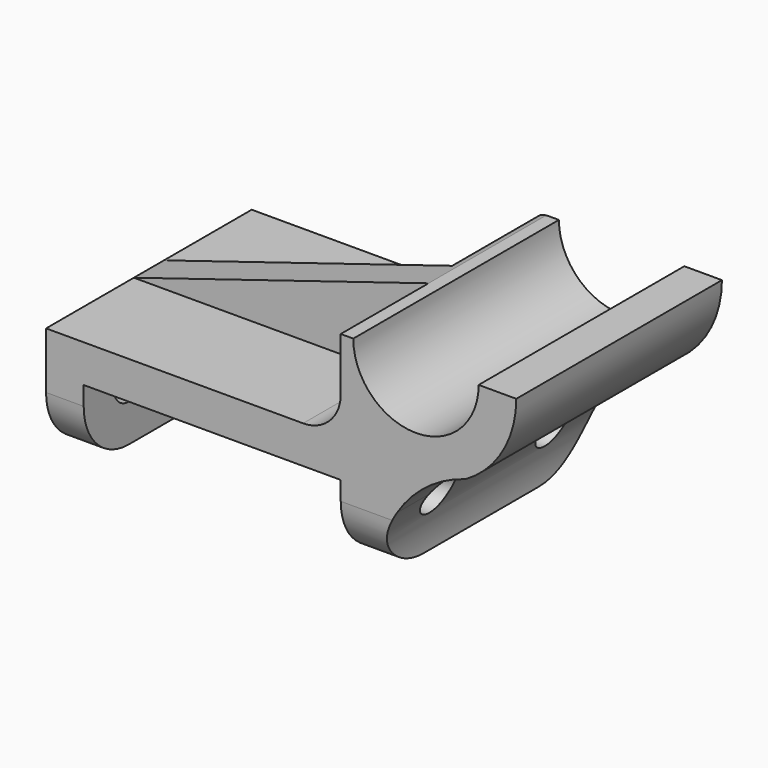
from build123d import *

# Parameters (mm, degrees)
F0_W      = 150
F0_H      = 65
F1_DEPTH  = 82
F10_W     = 82
F10_H     = 24
F2_DEPTH  = 82
F3_DEPTH  = 82
F4_DEPTH  = 82
F5_DEPTH  = 35
F7_DEPTH  = 35
F8_R      = 6
F12_R     = 6
F13_DEPTH = 150
F14_DEPTH = 150
F9_DEPTH  = 82


# Not quite as in the source:
# - a feature names something its author has since deleted; it is built from what else it names


with BuildPart() as f1:
    # F0 (on Front) → F1 (new body)
    with BuildSketch(Plane.XZ):
        with Locations((-16.9468223028, 32.5)):
            Rectangle(F0_W, F0_H)
    extrude(amount=F1_DEPTH)

    # F10 (on face) → F2 (cut)
    with BuildSketch(Plane.XZ.offset(82)):
        with BuildLine():
            ThreePointArc((20.002534413, 20.6353670047), (15.5702030299, 10.7379376133), (14.0531776972, 0))
            Line((14.0531776972, 0), (58.0531776972, 0))
            Line((58.0531776972, 0), (58.0531776972, 65))
            ThreePointArc((58.0531776972, 65), (53.7152597827, 48.9124515634), (41.8776017786, 37.1865571621))
            ThreePointArc((41.8776017786, 37.1865571621), (37.6930401765, 19.9858202792), (20.002534413, 20.6353670047))
        make_face()
        with Locations((-38.9468223028, 12)):
            Rectangle(F10_W, F10_H)
    extrude(amount=-F2_DEPTH, mode=Mode.SUBTRACT)

    # F11 (on face) → F3 (cut)
    with BuildSketch(Plane.XZ.offset(82)):
        Polygon((-91.9468223028, 36), (2.0531776972, 65), (-91.9468223028, 65), align=None)
    extrude(amount=-F3_DEPTH, mode=Mode.SUBTRACT)

    # F11 (on face) → F4 (cut)
    with BuildSketch(Plane.XZ.offset(82)):
        Polygon((-91.9468223028, 36), (2.0531776972, 65), (-91.9468223028, 65), align=None)
    extrude(amount=-F4_DEPTH, mode=Mode.SUBTRACT)

    # F11 (on face) → F5 (cut)
    with BuildSketch(Plane.XZ.offset(82)):
        with BuildLine():
            Line((2.0531776972, 48), (2.0531776972, 65))
            Line((2.0531776972, 65), (-91.9468223028, 36))
            Line((-91.9468223028, 36), (-9.9468223028, 36))
            ThreePointArc((-9.9468223028, 36), (-1.4615409285, 39.5147186258), (2.0531776972, 48))
        make_face()
    extrude(amount=-F5_DEPTH, mode=Mode.SUBTRACT)

    # F6 (on face) → F7 (cut)
    with BuildSketch(Plane(origin=(0, 0, 0), x_dir=(-1, 0, 0), z_dir=(0, 1, 0))):
        with BuildLine():
            Line((12, 36), (91.9468223028, 36))
            Line((91.9468223028, 36), (0, 64.3665728381))
            Line((0, 64.3665728381), (0, 48))
            ThreePointArc((0, 48), (3.5147186258, 39.5147186258), (12, 36))
        make_face()
    extrude(amount=-F7_DEPTH, mode=Mode.SUBTRACT)

    # F8 (on face) + F12 (on face) → F13 (cut)
    with BuildSketch(Plane(origin=(-91.9468223028, 0, 0), x_dir=(0, -1, 0), z_dir=(-1, 0, 0))):
        with Locations((18, 18)):
            Circle(F8_R)
        with Locations((64, 18)):
            Circle(F8_R)
    with BuildSketch(Plane(origin=(-91.9468223028, 0, 0), x_dir=(0, -1, 0), z_dir=(-1, 0, 0))):
        with Locations((18, 18)):
            Circle(F12_R)
    extrude(amount=-F13_DEPTH, mode=Mode.SUBTRACT)

    # F8 (on face) → F14 (cut)
    with BuildSketch(Plane(origin=(-91.9468223028, 0, 0), x_dir=(0, -1, 0), z_dir=(-1, 0, 0))):
        with BuildLine():
            Line((0, 0), (18, 0))
            ThreePointArc((18, 0), (5.2720779386, 5.2720779386), (0, 18))
            Line((0, 18), (0, 0))
        make_face()
        with BuildLine():
            ThreePointArc((82, 18), (76.7279220614, 5.2720779386), (64, 0))
            Line((64, 0), (82, 0))
            Line((82, 0), (82, 18))
        make_face()
    extrude(amount=-F14_DEPTH, mode=Mode.SUBTRACT)

    # F10 (on face) → F9 (cut)
    with BuildSketch(Plane.XZ.offset(82)):
        with BuildLine():
            ThreePointArc((41.8776017786, 37.1865571621), (29.4269949399, 30.9107323053), (20.002534413, 20.6353670047))
            ThreePointArc((20.002534413, 20.6353670047), (37.6930401765, 19.9858202792), (41.8776017786, 37.1865571621))
        make_face()
        with BuildLine():
            ThreePointArc((20.002534413, 20.6353670047), (15.5702030299, 10.7379376133), (14.0531776972, 0))
            Line((14.0531776972, 0), (58.0531776972, 0))
            Line((58.0531776972, 0), (58.0531776972, 65))
            ThreePointArc((58.0531776972, 65), (53.7152597827, 48.9124515634), (41.8776017786, 37.1865571621))
            ThreePointArc((41.8776017786, 37.1865571621), (37.6930401765, 19.9858202792), (20.002534413, 20.6353670047))
        make_face()
        with BuildLine():
            Line((46.0531776972, 65), (6.0531776972, 65))
            ThreePointArc((6.0531776972, 65), (12.5913823165, 50.2087841904), (27.9311842099, 45.0883679338))
            ThreePointArc((27.9311842099, 45.0883679338), (40.8443935069, 51.5382046192), (46.0531776972, 65))
        make_face()
    extrude(amount=-F9_DEPTH, mode=Mode.SUBTRACT)


solid = f1.part
